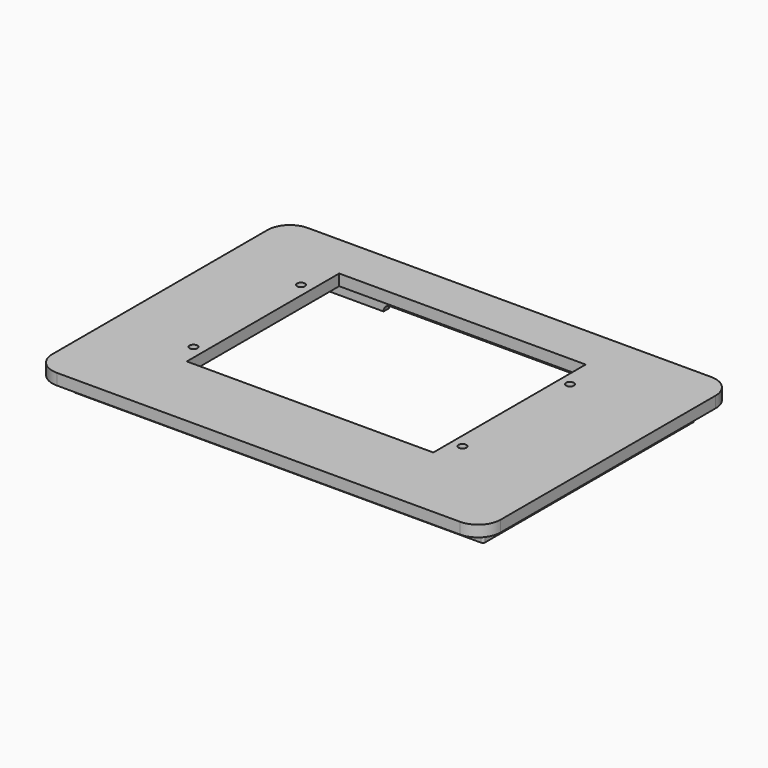
from build123d import *

# Parameters (mm, degrees)
F0_W     = 200
F0_H     = 140
F0_W_2   = 183
F0_H_2   = 118
F0_W_3   = 177
F0_H_3   = 112
F0_R     = 1.75
F0_W_4   = 110
F0_H_4   = 85
F1_DEPTH = 5
F2_DEPTH = 7.5
F3_R     = 10
F4_R     = 1
F5_R     = 2
F6_W     = 45
F6_H     = 3
F7_DEPTH = 25
F8_R     = 2.99999


# Not quite as in the source:
# - a fillet or chamfer is up to 0.001 mm smaller than in the source, because OpenCascade refuses the exact size


with BuildPart() as f1:
    # F0 (on Top) → F1 (new body)
    with BuildSketch(Plane.XY):
        Rectangle(F0_W, F0_H)
        Rectangle(F0_W_2, F0_H_2, mode=Mode.SUBTRACT)
        Rectangle(F0_W_2, F0_H_2)
        Rectangle(F0_W_3, F0_H_3, mode=Mode.SUBTRACT)
        Rectangle(F0_W_3, F0_H_3)
        with Locations((-65, -25)):
            Circle(F0_R, mode=Mode.SUBTRACT)
        with Locations((55, -25)):
            Circle(F0_R, mode=Mode.SUBTRACT)
        with Locations((-5, 7.5)):
            Rectangle(F0_W_4, F0_H_4, mode=Mode.SUBTRACT)
        with Locations((-65, 35)):
            Circle(F0_R, mode=Mode.SUBTRACT)
        with Locations((55, 35)):
            Circle(F0_R, mode=Mode.SUBTRACT)
    extrude(amount=F1_DEPTH)

    # F0 (on Top) → F2 (join)
    with BuildSketch(Plane.XY):
        Rectangle(F0_W_2, F0_H_2)
        Rectangle(F0_W_3, F0_H_3, mode=Mode.SUBTRACT)
    extrude(amount=-F2_DEPTH)

    # F3
    f3_edges = [f1.edges().sort_by_distance(p)[0] for p in [
        (-100, 70, 2.5),
        (-100, -70, 2.5),
        (100, -70, 2.5),
        (100, 70, 2.5),
    ]]
    fillet(f3_edges, radius=F3_R)

    # F4
    f4_edges = [f1.edges().sort_by_distance(p)[0] for p in [
        (-91.5, -59, -3.75),
        (91.5, -59, -3.75),
        (-91.5, 59, -3.75),
        (91.5, 59, -3.75),
    ]]
    fillet(f4_edges, radius=F4_R)

    # F5
    f5_edges = [f1.edges().sort_by_distance(p)[0] for p in [
        (-66.75, -25, 0),
        (53.25, -25, 0),
        (-66.75, 35, 0),
        (53.25, 35, 0),
    ]]
    fillet(f5_edges, radius=F5_R)

    # F6 (on face) → F7 (cut)
    with BuildSketch(Plane(origin=(0, 59, 0), x_dir=(-1, 0, 0), z_dir=(0, 1, 0))):
        with Locations((-22.5, -6)):
            Rectangle(F6_W, F6_H)
        with Locations((22.5, -6)):
            Rectangle(F6_W, F6_H)
    extrude(amount=-F7_DEPTH, mode=Mode.SUBTRACT)

    # F8 (radius 3 in the source; OpenCascade refuses exactly that, so slightly less here)
    f8_edges = [f1.edges().sort_by_distance(p)[0] for p in [
        (-45, 57.5, -4.5),
        (45, 57.5, -4.5),
    ]]
    fillet(f8_edges, radius=F8_R)


solid = f1.part
